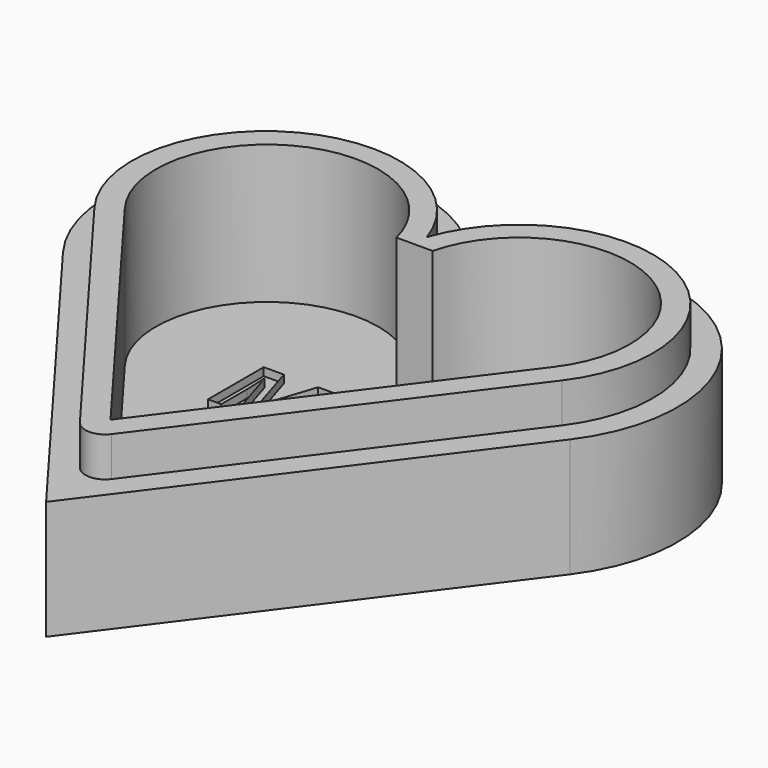
from build123d import *

# Parameters (mm, degrees)
F1_DEPTH     = 10
F2_DEPTH     = 30
F4_DEPTH     = 35
F5_TEXT_SIZE = 24.6429570123
F6_DEPTH     = 2
F7_R         = 5


# Not quite as in the source:
# - Text() gives the source's letters only with a copy of the font that has no kerning and outlines rounded to 1/6400 em; it was checked with that copy


with BuildPart() as f1:
    # F0 (on Top) → F1 (new body)
    with BuildSketch(Plane.XY):
        with BuildLine():
            Line((-59.0400012048, 11.2256030415), (0, -67.4944030271))
            Line((0, -67.4944030271), (59.0400012048, 11.2256030415))
            ThreePointArc((59.0400012048, 11.2256030415), (47.7776343081, 61.3971776448), (0, 42.388614674))
            ThreePointArc((0, 42.388614674), (-47.7776343081, 61.3971776448), (-59.0400012048, 11.2256030415))
        make_face()
    extrude(amount=F1_DEPTH)

    # F0 (on Top) → F2 (join)
    with BuildSketch(Plane.XY):
        with BuildLine():
            Line((-64.000001306, 7.5056031764), (0, -77.8277367353))
            Line((0, -77.8277367353), (64.000001306, 7.5056031764))
            ThreePointArc((64.000001306, 7.5056031764), (55.9999997823, 63.5056029588), (0, 55.5056014351))
            ThreePointArc((0, 55.5056014351), (-55.9999997823, 63.5056029588), (-64.000001306, 7.5056031764))
        make_face()
        with BuildLine():
            Line((59.0400012048, 11.2256030415), (0, -67.4944030271))
            Line((0, -67.4944030271), (-59.0400012048, 11.2256030415))
            ThreePointArc((-59.0400012048, 11.2256030415), (-47.7776343081, 61.3971776448), (0, 42.388614674))
            ThreePointArc((0, 42.388614674), (47.7776343081, 61.3971776448), (59.0400012048, 11.2256030415))
        make_face(mode=Mode.SUBTRACT)
        with BuildLine():
            Line((-59.0400012048, 11.2256030415), (0, -67.4944030271))
            Line((0, -67.4944030271), (59.0400012048, 11.2256030415))
            ThreePointArc((59.0400012048, 11.2256030415), (47.7776343081, 61.3971776448), (0, 42.388614674))
            ThreePointArc((0, 42.388614674), (-47.7776343081, 61.3971776448), (-59.0400012048, 11.2256030415))
        make_face()
    extrude(amount=-F2_DEPTH)

    # F3 (on face) → F4 (cut)
    with BuildSketch(Plane.XY.offset(10)):
        with BuildLine():
            Line((-54.2400011068, 14.8256029109), (0, -57.4944026644))
            Line((0, -57.4944026644), (54.2400011068, 14.8256029109))
            ThreePointArc((54.2400011068, 14.8256029109), (43.8519793856, 57.0101600273), (4.5554236943, 38.4837311975))
            Line((4.5554236943, 38.4837311975), (0, 38.4837311975))
            Line((0, 38.4837311975), (-4.5554236943, 38.4837311975))
            ThreePointArc((-4.5554236943, 38.4837311975), (-43.8519793856, 57.0101600273), (-54.2400011068, 14.8256029109))
        make_face()
    extrude(amount=-F4_DEPTH, mode=Mode.SUBTRACT)

    # F5 (on face) → F6 (join)
    with BuildSketch(Plane.XY.offset(-25)):
        with Locations((-32.2399186037, 10.8283823356)):
            Text('MUM', F5_TEXT_SIZE, font='Open Sans', font_style=FontStyle.BOLD, text_align=(TextAlign.LEFT, TextAlign.BOTTOM))
    extrude(amount=F6_DEPTH)

    # F7
    f7_edges = [f1.edges().sort_by_distance(p)[0] for p in [
        (0, -67.494403, 5),
    ]]
    fillet(f7_edges, radius=F7_R)


solid = f1.part
